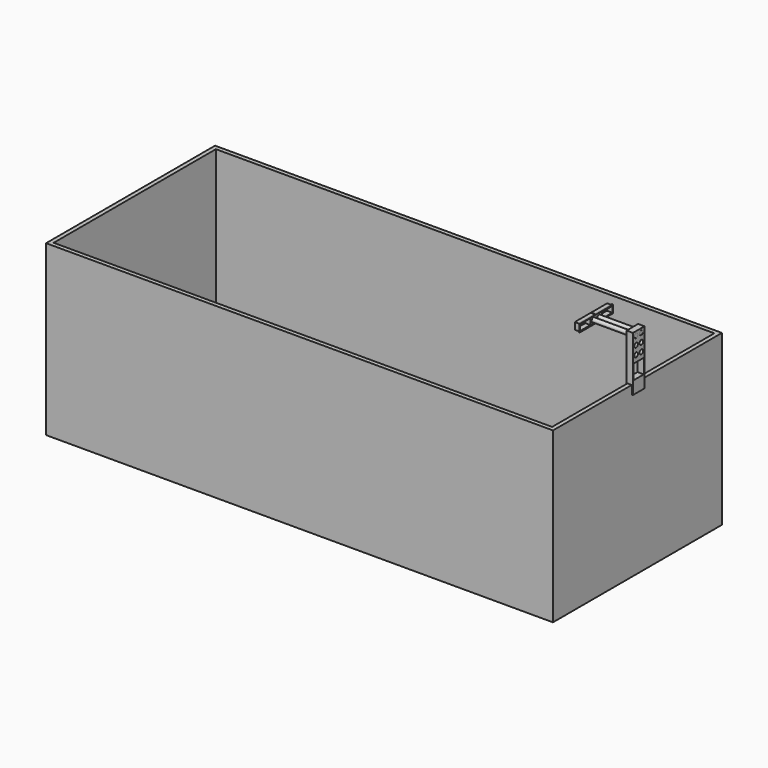
from build123d import *

# Parameters (mm, degrees)
F0_W          = 1.5
F0_H          = 1
F0_H_2        = 16
F0_R          = 5.25
F0_W_2        = 30
F0_H_3        = 14
F1_DEPTH      = 3
F2_DEPTH      = 10
F2_DEPTH_BACK = 2
F5_W          = 1200
F5_H          = 500
F5_W_2        = 1180
F5_H_2        = 480
F6_DEPTH      = 400
F7_W          = 10
F7_H          = 2
F7_W_2        = 1
F7_H_2        = 30
F8_DEPTH      = 10
F9_DEPTH      = 20
F10_R         = 5.25
F11_DEPTH     = 15
F12_W         = 110
F12_H         = 5


# Not quite as in the source:
# - a feature names something its author has since deleted; it is built from what else it names
# - the program builds the solid bodies; features that only make, move or delete a surface that nothing else refers to are left out


with BuildPart() as f1:
    # F0 (on Right) → F1 (new body)
    with BuildSketch(Plane.YZ):
        Polygon((-0.75, 9), (-49.5, 9), (-49.5, -9), (-0.75, -9), (-0.75, -8), (-13, -8), (-16, -8), (-48, -8), (-48, 8), (-16, 8), (-13, 8), (-0.75, 8), align=None)
        with Locations((0, 8.5)):
            Rectangle(F0_W, F0_H)
        Polygon((49.5, 9), (0.75, 9), (0.75, 8), (13, 8), (16, 8), (48, 8), (48, -8), (16, -8), (13, -8), (0.75, -8), (0.75, -9), (49.5, -9), align=None)
        with Locations((0, -8.5)):
            Rectangle(F0_W, F0_H)
        Rectangle(F0_W, F0_H_2)
        Polygon((13, 8), (0.75, 8), (0.75, -8), (13, -8), (16, -8), (48, -8), (48, 8), (16, 8), align=None)
        with Locations((7.75, 0)):
            Circle(F0_R, mode=Mode.SUBTRACT)
        with Locations((32, 0)):
            Rectangle(F0_W_2, F0_H_3, mode=Mode.SUBTRACT)
    extrude(amount=F1_DEPTH)

    # F0 (on Right) → F2 (join, two sides)
    with BuildSketch(Plane.YZ) as f2_sk:
        Polygon((-0.75, -8), (-0.75, 8), (-13, 8), (-16, 8), (-48, 8), (-48, -8), (-16, -8), (-13, -8), align=None)
        with Locations((-32, 0)):
            Rectangle(F0_W_2, F0_H_3, mode=Mode.SUBTRACT)
        with Locations((-7.75, 0)):
            Circle(F0_R, mode=Mode.SUBTRACT)
        Polygon((13, 8), (0.75, 8), (0.75, -8), (13, -8), (16, -8), (48, -8), (48, 8), (16, 8), align=None)
        with Locations((7.75, 0)):
            Circle(F0_R, mode=Mode.SUBTRACT)
        with Locations((32, 0)):
            Rectangle(F0_W_2, F0_H_3, mode=Mode.SUBTRACT)
    extrude(amount=-F2_DEPTH)
    extrude(f2_sk.sketch, amount=F2_DEPTH_BACK)


with BuildPart() as f6:
    # F5 (on offset) → F6 (new body)
    with BuildSketch(Plane.XY.offset(-500)):
        with Locations((-500, 0)):
            Rectangle(F5_W, F5_H)
        with Locations((-500, 0)):
            Rectangle(F5_W_2, F5_H_2, mode=Mode.SUBTRACT)
    extrude(amount=F6_DEPTH)


with BuildPart() as f8:
    # F7 (on face) → F8 (new body)
    with BuildSketch(Plane.XY.offset(-100)):
        Polygon((101, 17), (101, 15), (101, -15), (101, -17), (103, -17), (103, 17), align=None)
        Polygon((90, -15), (90, 15), (90, 17), (88, 17), (88, -17), (90, -17), align=None)
        with Locations((95, 16)):
            Rectangle(F7_W, F7_H)
        with Locations((100.5, 16)):
            Rectangle(F7_W_2, F7_H)
        with Locations((100.5, -16)):
            Rectangle(F7_W_2, F7_H)
        with Locations((95, -16)):
            Rectangle(F7_W, F7_H)
        with Locations((100.5, 0)):
            Rectangle(F7_W_2, F7_H_2)
        with Locations((95, 0)):
            Rectangle(F7_W, F7_H_2)
    extrude(amount=F8_DEPTH)

    # F7 (on face) → F9 (join)
    with BuildSketch(Plane.XY.offset(-100)):
        Polygon((90, -15), (90, 15), (90, 17), (88, 17), (88, -17), (90, -17), align=None)
        Polygon((101, 17), (101, 15), (101, -15), (101, -17), (103, -17), (103, 17), align=None)
    extrude(amount=-F9_DEPTH)

    # F10 (on face) → F11 (join)
    with BuildSketch(Plane.YZ.offset(103)):
        Polygon((-15, -90), (-17, -90), (-17, -100), (17, -100), (17, -90), (15, -90), align=None)
        Polygon((-17, 9.5), (-17, -90), (-15, -90), (-15, -55.25), (15, -55.25), (15, -90), (17, -90), (17, 9.5), align=None)
        with Locations((-7.75, -40)):
            Circle(F10_R, mode=Mode.SUBTRACT)
        with Locations((-7.75, -20)):
            Circle(F10_R, mode=Mode.SUBTRACT)
        with Locations((-7.75, 0)):
            Circle(F10_R, mode=Mode.SUBTRACT)
        with Locations((7.75, -40)):
            Circle(F10_R, mode=Mode.SUBTRACT)
        with Locations((7.75, -20)):
            Circle(F10_R, mode=Mode.SUBTRACT)
        with Locations((7.75, 0)):
            Circle(F10_R, mode=Mode.SUBTRACT)
    extrude(amount=-F11_DEPTH)


with BuildPart() as f13:
    # F12 (on Top) → F13 (revolve)
    with BuildSketch(Plane.XY):
        with Locations((48, -5)):
            Rectangle(F12_W, F12_H)
    revolve(axis=Axis((48, -7.5, 0), (1, 0, 0)))


with BuildPart() as f14:
    # F12 (on Top) → F14 (revolve)
    with BuildSketch(Plane.XY):
        with Locations((48, 5)):
            Rectangle(F12_W, F12_H)
    revolve(axis=Axis((48, 7.5, 0), (1, 0, 0)))


solid = Compound([f1.part, f6.part, f8.part, f13.part, f14.part])
